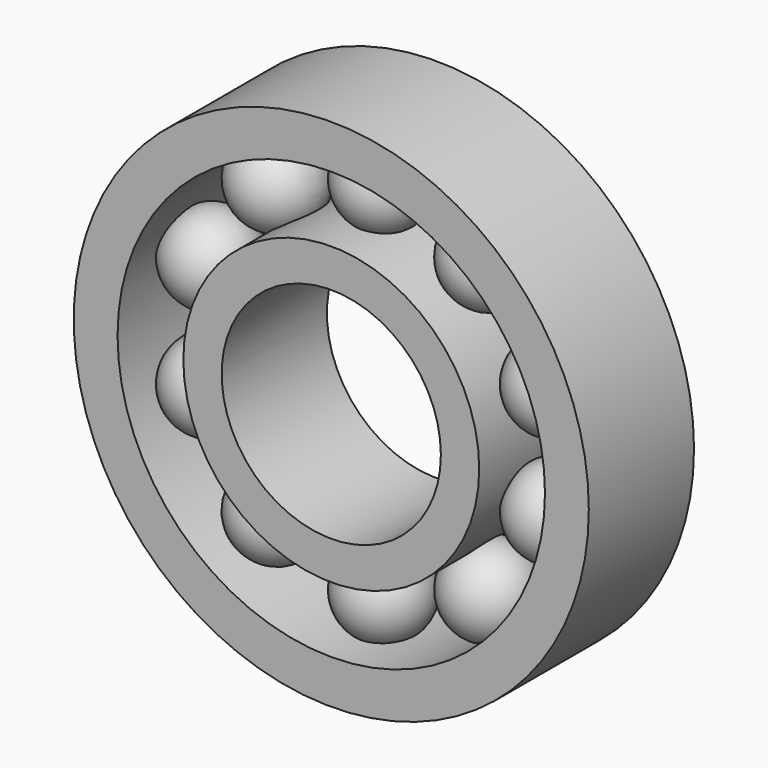
from build123d import *

# Parameters (mm, degrees)
F0_R     = 13.5
F0_R_2   = 10
F1_DEPTH = 6
F2_R     = 23.5
F2_R_2   = 19.5
F3_DEPTH = 6
F7_COUNT = 10


with BuildPart() as f1:
    # F0 (on Front) → F1 (new body, symmetric)
    with BuildSketch(Plane.XZ):
        Circle(F0_R)
        Circle(F0_R_2, mode=Mode.SUBTRACT)
    extrude(amount=F1_DEPTH, both=True)


with BuildPart() as f3:
    # F2 (on Front) → F3 (new body, symmetric)
    with BuildSketch(Plane.XZ):
        Circle(F2_R)
        Circle(F2_R_2, mode=Mode.SUBTRACT)
    extrude(amount=F3_DEPTH, both=True)


with BuildPart() as f5:
    # F4 (on Front) → F5 (revolve)
    with BuildSketch(Plane.XZ):
        with BuildLine():
            Line((0, 20.5), (0, 12.5))
            ThreePointArc((0, 12.5), (4, 16.5), (0, 20.5))
        make_face()
    revolve(axis=Axis((0, 0, 16.5), (0, 0, -1)))


with BuildPart() as f7_1:
    # F7: instance of F5
    add(f5.part.rotate(Axis((0, 5.8803767897, 0), (0, 1, 0)), 1 * 360 / F7_COUNT))


with BuildPart() as f7_2:
    # F7: instance of F5
    add(f5.part.rotate(Axis((0, 5.8803767897, 0), (0, 1, 0)), 2 * 360 / F7_COUNT))


with BuildPart() as f7_3:
    # F7: instance of F5
    add(f5.part.rotate(Axis((0, 5.8803767897, 0), (0, 1, 0)), 3 * 360 / F7_COUNT))


with BuildPart() as f7_4:
    # F7: instance of F5
    add(f5.part.rotate(Axis((0, 5.8803767897, 0), (0, 1, 0)), 4 * 360 / F7_COUNT))


with BuildPart() as f7_5:
    # F7: instance of F5
    add(f5.part.rotate(Axis((0, 5.8803767897, 0), (0, 1, 0)), 5 * 360 / F7_COUNT))


with BuildPart() as f7_6:
    # F7: instance of F5
    add(f5.part.rotate(Axis((0, 5.8803767897, 0), (0, 1, 0)), 6 * 360 / F7_COUNT))


with BuildPart() as f7_7:
    # F7: instance of F5
    add(f5.part.rotate(Axis((0, 5.8803767897, 0), (0, 1, 0)), 7 * 360 / F7_COUNT))


with BuildPart() as f7_8:
    # F7: instance of F5
    add(f5.part.rotate(Axis((0, 5.8803767897, 0), (0, 1, 0)), 8 * 360 / F7_COUNT))


with BuildPart() as f7_9:
    # F7: instance of F5
    add(f5.part.rotate(Axis((0, 5.8803767897, 0), (0, 1, 0)), 9 * 360 / F7_COUNT))


solid = Compound([f1.part, f3.part, f5.part, f7_1.part, f7_2.part, f7_3.part, f7_4.part, f7_5.part, f7_6.part, f7_7.part, f7_8.part, f7_9.part])
